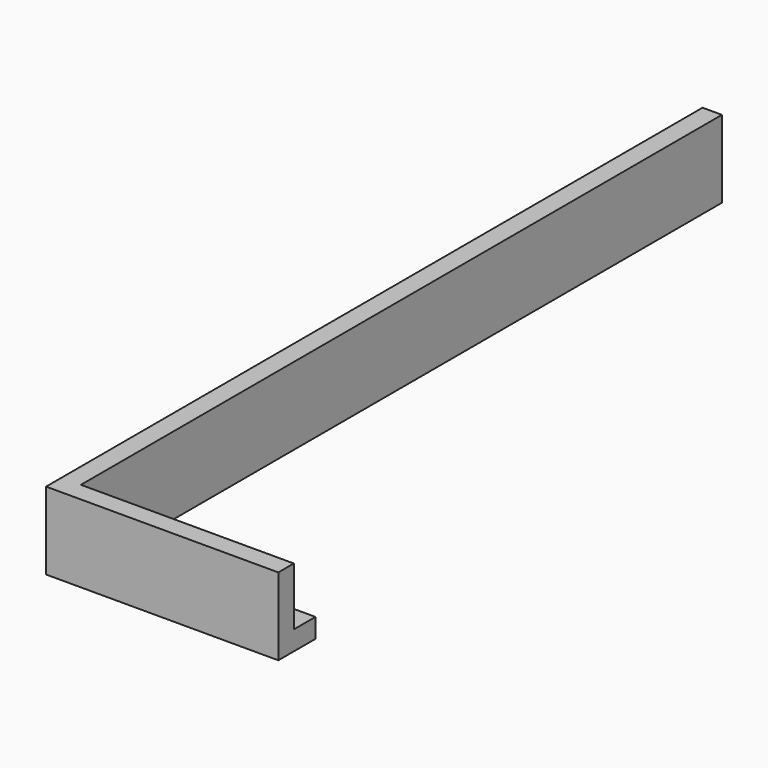
from build123d import *

# Parameters (mm, degrees)
F0_W     = 3.175
F0_H     = 127
F0_H_2   = 4.445
F0_H_3   = 3.175
F0_W_2   = 34.925
F1_DEPTH = 12.7
F2_DEPTH = 3.175


# Not quite as in the source:
# - a length typed as a fraction of an inch, garbled in the dataset ("3 / 203.2 mm" for 3/8 in), is restored


with BuildPart() as f1:
    # F0 (on Top) → F1 (new body)
    with BuildSketch(Plane.XY):
        with Locations((-1.5875, 63.5)):
            Rectangle(F0_W, F0_H)
        with Locations((-1.5875, -2.2225)):
            Rectangle(F0_W, F0_H_2)
        with Locations((-1.5875, -6.0325)):
            Rectangle(F0_W, F0_H_3)
        with Locations((17.4625, -6.0325)):
            Rectangle(F0_W_2, F0_H_3)
    extrude(amount=F1_DEPTH)

    # F0 (on Top) → F2 (join)
    with BuildSketch(Plane.XY):
        with Locations((17.4625, -2.2225)):
            Rectangle(F0_W_2, F0_H_2)
    extrude(amount=F2_DEPTH)


solid = f1.part
